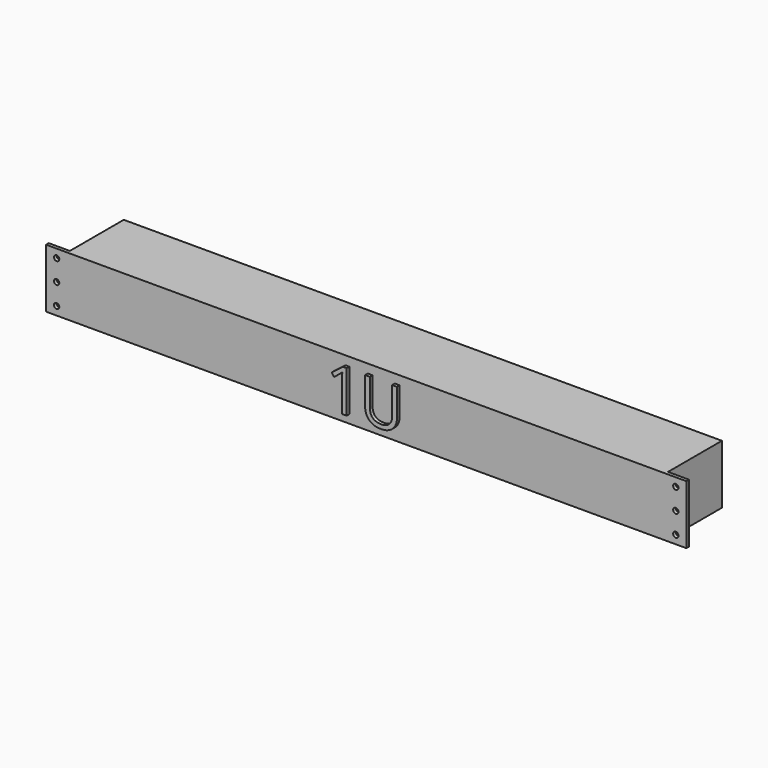
from build123d import *

# Parameters (mm, degrees)
F0_W         = 482.6
F0_H         = 44.45
F1_DEPTH     = 2.54
F2_W         = 450.85
F2_H         = 44.45
F3_DEPTH     = 50.8
F5_D         = 4.0386
F6_TEXT_SIZE = 44.0972222222
F7_DEPTH     = 2.54


# Not quite as in the source:
# - Text() gives the source's letters only with a copy of the font that has no kerning and outlines rounded to 1/6400 em; it was checked with that copy


with BuildPart() as f1:
    # F0 (on Front) → F1 (new body)
    with BuildSketch(Plane.XZ):
        Rectangle(F0_W, F0_H)
    extrude(amount=F1_DEPTH)

    # F2 (on face) → F3 (join)
    with BuildSketch(Plane(origin=(0, 0, 0), x_dir=(-1, 0, 0), z_dir=(0, 1, 0))):
        Rectangle(F2_W, F2_H)
    extrude(amount=F3_DEPTH)

    # F5 (through all)
    with Locations(Plane.XZ.offset(2.54)):
        with Locations((-233.3625, -44.45), (-233.3625, -60.325), (233.3625, 15.875), (233.3625, -28.575), (233.3625, -44.45), (233.3625, 0), (233.3625, -60.325), (233.3625, -15.875), (-233.3625, 15.875), (-233.3625, 0), (-233.3625, -15.875), (-233.3625, -28.575)):
            Hole(F5_D / 2)

    # F6 (on face) → F7 (join)
    with BuildSketch(Plane.XZ.offset(2.54)):
        with Locations((-28.0844184028, -15.875)):
            Text('1U', F6_TEXT_SIZE, font='Open Sans', text_align=(TextAlign.LEFT, TextAlign.BOTTOM))
    extrude(amount=F7_DEPTH)


solid = f1.part
